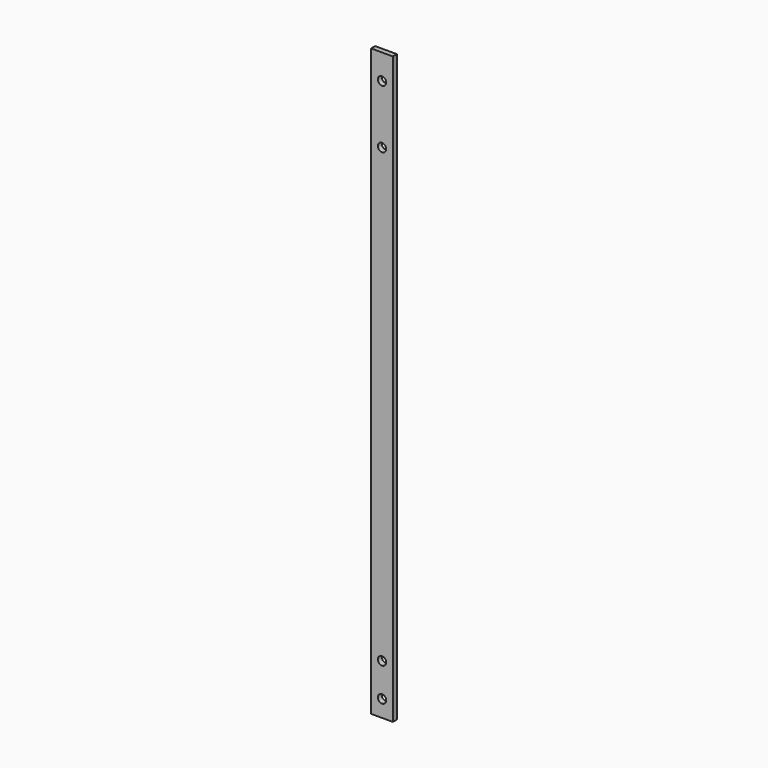
from build123d import *

# Parameters (mm, degrees)
F0_W     = 13
F0_H     = 350
F1_DEPTH = 3
F3_DEPTH = 3
F5_DEPTH = 25
F7_DEPTH = 25
F8_DEPTH = 25


with BuildPart() as f1:
    # F0 (on Front) → F1 (new body)
    with BuildSketch(Plane.XZ):
        Rectangle(F0_W, F0_H)
    extrude(amount=F1_DEPTH)

    # F2 (on face) → F3 (cut)
    with BuildSketch(Plane.XZ.offset(3)):
        with BuildLine():
            ThreePointArc((2.5, 160), (1.767766953, 161.767766953), (0, 162.5))
            ThreePointArc((0, 162.5), (-1.767766953, 158.232233047), (2.5, 160))
        make_face()
    extrude(amount=-F3_DEPTH, mode=Mode.SUBTRACT)

    # F4 (on face) → F5 (cut)
    with BuildSketch(Plane.XZ.offset(3)):
        with BuildLine():
            ThreePointArc((2.5, -145), (-1.767766953, -143.232233047), (0, -147.5))
            ThreePointArc((0, -147.5), (1.767766953, -146.767766953), (2.5, -145))
        make_face()
    extrude(amount=-F5_DEPTH, mode=Mode.SUBTRACT)

    # F6 (on face) → F7 (cut)
    with BuildSketch(Plane.XZ.offset(3)):
        with BuildLine():
            ThreePointArc((2.5, 125), (1.767766953, 126.767766953), (0, 127.5))
            ThreePointArc((0, 127.5), (-1.767766953, 123.232233047), (2.5, 125))
        make_face()
    extrude(amount=-F7_DEPTH, mode=Mode.SUBTRACT)

    # F4 (on face) → F8 (cut)
    with BuildSketch(Plane.XZ.offset(3)):
        with BuildLine():
            ThreePointArc((0, -162.5), (-2.5, -165), (0, -167.5))
            Line((0, -167.5), (0, -165))
            Line((0, -165), (0, -162.5))
        make_face()
        with BuildLine():
            ThreePointArc((2.5, -145), (-1.767766953, -143.232233047), (0, -147.5))
            ThreePointArc((0, -147.5), (1.767766953, -146.767766953), (2.5, -145))
        make_face()
        with BuildLine():
            Line((0, -165), (0, -167.5))
            ThreePointArc((0, -167.5), (1.767766953, -166.767766953), (2.5, -165))
            ThreePointArc((2.5, -165), (1.767766953, -163.232233047), (0, -162.5))
            Line((0, -162.5), (0, -165))
        make_face()
    extrude(amount=-F8_DEPTH, mode=Mode.SUBTRACT)


solid = f1.part
